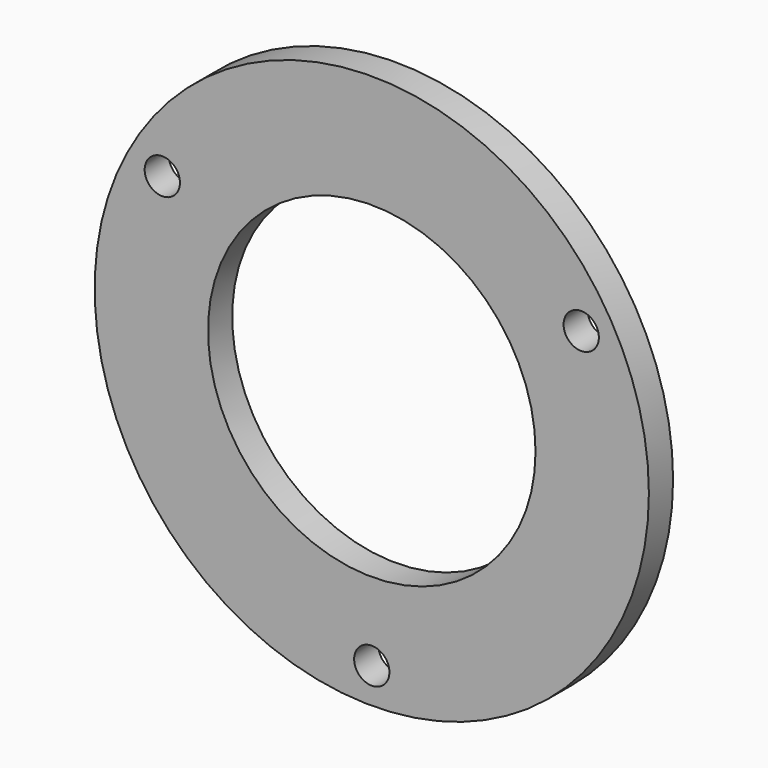
from build123d import *

# Parameters (mm, degrees)
F0_R            = 55
F0_R_2          = 32.5
F1_DEPTH        = 3
F2_R            = 3.5
F3_DEPTH        = 12.5
F3_COPIES_COUNT = 3
F4_R            = 4.5
F5_DEPTH        = 12.5


# Not quite as in the source:
# - a pattern or mirror of a feature is missing from the dataset's text; its kind, count and spacing are read off the source's solid


with BuildPart() as f1:
    # F0 (on Front) → F1 (new body, symmetric)
    with BuildSketch(Plane.XZ):
        Circle(F0_R)
        Circle(F0_R_2, mode=Mode.SUBTRACT)
    extrude(amount=F1_DEPTH, both=True)

    # F2 (on Front) → F3 (cut, symmetric)
    with BuildSketch(Plane.XZ):
        with Locations((0, -48)):
            Circle(F2_R)
    f3 = extrude(amount=F3_DEPTH, both=True, mode=Mode.SUBTRACT)

    # F3_copies: F3 ×3 about axis
    f3_copies_axis = Axis((0, 0, 0), (0, 1, 0))
    for i in range(1, F3_COPIES_COUNT):
        add(f3.rotate(f3_copies_axis, i * 360 / F3_COPIES_COUNT), mode=Mode.SUBTRACT)

    # F4 (on Front) → F5 (cut, symmetric)
    with BuildSketch(Plane.XZ):
        with Locations((15.9173712738, 59.4044383168)):
            Circle(F4_R)
    extrude(amount=F5_DEPTH, both=True, mode=Mode.SUBTRACT)


solid = f1.part
